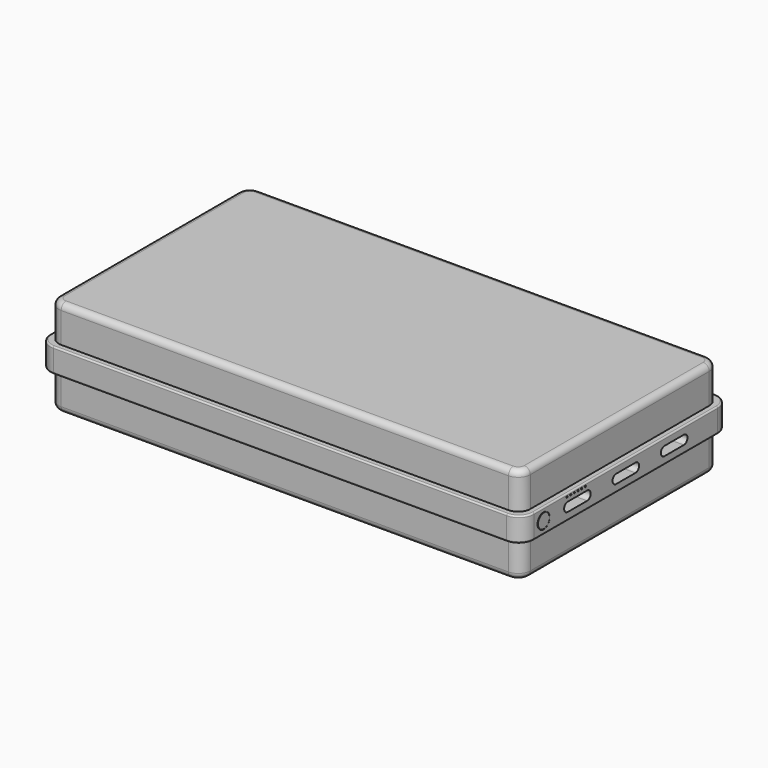
from build123d import *

# Parameters (mm, degrees)
F0_W        = 80
F0_H        = 43
F1_DEPTH    = 4
F2_W        = 78
F2_H        = 41
F3_DEPTH    = 12
F4_R        = 5
F5_R        = 0.5
F6_R        = 2
F7_T1_DEPTH = 12
F7_T4_ANGLE = 90
F11_R       = 2.5
F12_DEPTH   = 0.25
F13_DEPTH   = 5
F14_R       = 2.375
F15_DEPTH   = 0.3
F16_R       = 0.25
F17_DEPTH   = 0.5


# Not quite as in the source:
# - a fillet or chamfer that OpenCascade refuses, or shapes differently, is made with other operations: its cross-section is extruded or revolved along the edge and cut away or added


with BuildPart() as f1:
    # F0 (on Top) → F1 (new body)
    with BuildSketch(Plane.XY):
        with Locations((40, 21.5)):
            Rectangle(F0_W, F0_H)
    extrude(amount=F1_DEPTH)

    # F2 (on face) → F3 (join)
    with BuildSketch(Plane.XY.offset(4)):
        with Locations((39, 20.5)):
            Rectangle(F2_W, F2_H)
    extrude(amount=F3_DEPTH)

    # F4
    f4_edges = [f1.edges().sort_by_distance(p)[0] for p in [
        (80, 43, 2),
    ]]
    fillet(f4_edges, radius=F4_R)

    # F5
    f5_edges = [f1.edges().sort_by_distance(p)[0] for p in [
        (37.5, 43, 4),
        (78.535534, 41.535534, 4),
        (80, 19, 4),
    ]]
    fillet(f5_edges, radius=F5_R)

    # F6
    f6_edges = [f1.edges().sort_by_distance(p)[0] for p in [
        (78, 20.5, 16),
        (39, 41, 16),
    ]]
    fillet(f6_edges, radius=F6_R)

    # F7: fillet of radius 4 on 1 edges, made by hand

    # F7_s2 → F7_t1 (cut)
    with BuildSketch(Plane.XY.offset(4)):
        with BuildLine():
            ThreePointArc((74, 41), (76.8284271247, 39.8284271247), (78, 37))
            Line((78, 37), (78, 41))
            Line((78, 41), (74, 41))
        make_face()
    extrude(amount=F7_T1_DEPTH, mode=Mode.SUBTRACT)

    # F7_s3 → F7_t4 (revolve, cut)
    with BuildSketch(Plane.XZ.offset(-37)):
        with BuildLine():
            ThreePointArc((76, 16), (77.4142135624, 15.4142135624), (78, 14))
            Line((78, 14), (78, 16))
            Line((78, 16), (76, 16))
        make_face()
    revolve(axis=Axis((74, 37, 16), (0, 0, 1)), revolution_arc=F7_T4_ANGLE, mode=Mode.SUBTRACT)

    # F8: F1 across face


with BuildPart() as f1_1:
    add(f1.part)
    add(f1.part.mirror(Plane(origin=(39.2268461901, 0, 7.956765433), x_dir=(1, 0, 0), z_dir=(0, -1, 0))))

    # F9: F1 across face


with BuildPart() as f1_2:
    add(f1_1.part)
    add(f1_1.part.mirror(Plane(origin=(0, 0, 7.9181659321), x_dir=(0, -1, 0), z_dir=(-1, 0, 0))))

    # F10: F1 across face


with BuildPart() as f1_3:
    add(f1_2.part)
    add(f1_2.part.mirror(Plane(origin=(0, 0, 0), x_dir=(1, 0, 0), z_dir=(0, 0, -1))))

    # F11 (on face) → F12 (cut)
    with BuildSketch(Plane.YZ.offset(80)):
        with Locations((-34, 0)):
            Circle(F11_R)
    extrude(amount=-F12_DEPTH, mode=Mode.SUBTRACT)

    # F11 (on face) → F13 (cut)
    with BuildSketch(Plane.YZ.offset(80)):
        with BuildLine():
            Line((-24, -1.5), (-16, -1.5))
            ThreePointArc((-16, -1.5), (-14.5, 0), (-16, 1.5))
            Line((-16, 1.5), (-24, 1.5))
            ThreePointArc((-24, 1.5), (-25.5, 0), (-24, -1.5))
        make_face()
        with BuildLine():
            Line((-4, -1.5), (4, -1.5))
            ThreePointArc((4, -1.5), (5.5, 0), (4, 1.5))
            Line((4, 1.5), (-4, 1.5))
            ThreePointArc((-4, 1.5), (-5.5, 0), (-4, -1.5))
        make_face()
        with BuildLine():
            Line((16, -1.5), (24, -1.5))
            ThreePointArc((24, -1.5), (25.5, 0), (24, 1.5))
            Line((24, 1.5), (16, 1.5))
            ThreePointArc((16, 1.5), (14.5, 0), (16, -1.5))
        make_face()
    extrude(amount=-F13_DEPTH, mode=Mode.SUBTRACT)

    # F14 (on face) → F15 (join)
    with BuildSketch(Plane.YZ.offset(79.75)):
        with Locations((-34, 0)):
            Circle(F14_R)
    extrude(amount=F15_DEPTH)

    # F16 (on face) → F17 (cut)
    with BuildSketch(Plane.YZ.offset(80)):
        with Locations((-21.2721988683, 3)):
            Circle(F16_R)
        with Locations((-18.2721988683, 3)):
            Circle(F16_R)
        with Locations((-16.7721988683, 3)):
            Circle(F16_R)
        with Locations((-22.7721988683, 3)):
            Circle(F16_R)
        with Locations((-24.2721988683, 3)):
            Circle(F16_R)
        with Locations((-19.7721988683, 3)):
            Circle(F16_R)
    extrude(amount=-F17_DEPTH, mode=Mode.SUBTRACT)


solid = f1_3.part
